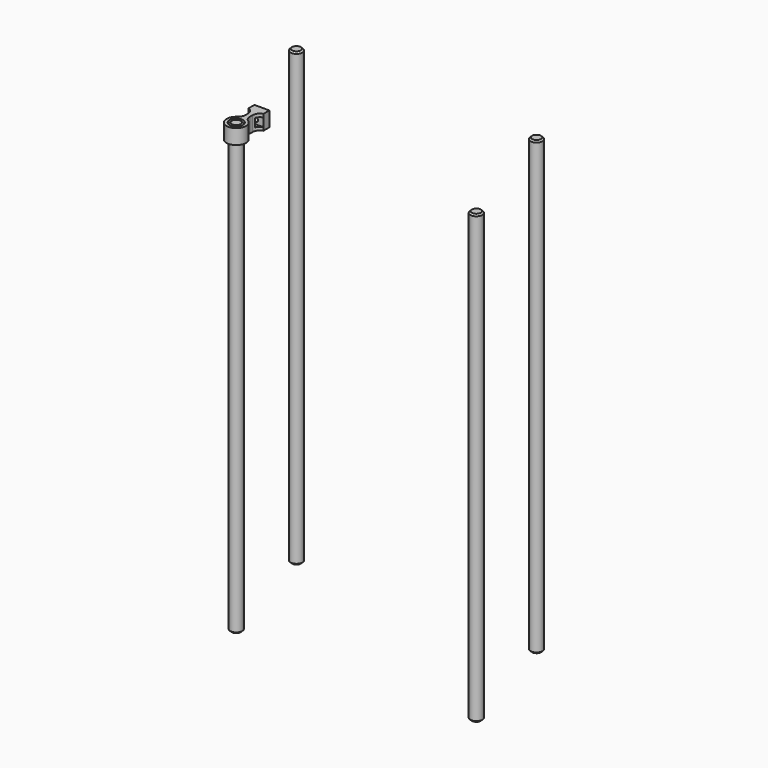
from build123d import *

# Parameters (mm, degrees)
F0_R          = 4
F1_DEPTH      = 303
F2_SIZE       = 1
F2_2_SIZE     = 1
F3_R          = 4
F4_DEPTH      = 280
F4_DEPTH_BACK = 20
F5_SIZE       = 1
F5_2_SIZE     = 1
F6_R          = 4.5
F7_DEPTH      = 10
F9_W          = 3
F9_H          = 5.7
F10_DEPTH     = 3
F8_R          = 1.5
F11_DEPTH     = 7
F12_T1_DEPTH  = 2.15
F12_T3_DEPTH  = 10
F12_T8_DEPTH  = 25.9984800354
F12_T15_DEPTH = 25.9984800354
F12_T21_DEPTH = 25.9984800354
F12_T28_DEPTH = 25.9984800354


# Not quite as in the source:
# - a fillet or chamfer that OpenCascade refuses, or shapes differently, is made with other operations: its cross-section is extruded or revolved along the edge and cut away or added


with BuildPart() as f1:
    # F0 (on Top) → F1 (new body)
    with BuildSketch(Plane.XY):
        with Locations((-80.5, 0)):
            Circle(F0_R)
    extrude(amount=F1_DEPTH)

    # F2
    f2_edges = [f1.edges().sort_by_distance(p)[0] for p in [
        (-84.5, 0, 0),
        (-84.5, 0, 303),
    ]]
    chamfer(f2_edges, length=F2_SIZE)


with BuildPart() as f1b:
    # F0 (on Top) → F1, piece 2 (new body)
    with BuildSketch(Plane.XY):
        with Locations((80.5, 0)):
            Circle(F0_R)
    extrude(amount=F1_DEPTH)

    # F2#2
    f2_2_edges = [f1b.edges().sort_by_distance(p)[0] for p in [
        (76.5, 0, 0),
        (76.5, 0, 303),
    ]]
    chamfer(f2_2_edges, length=F2_2_SIZE)


with BuildPart() as f4:
    # F3 (on Top) → F4 (new body, two sides)
    with BuildSketch(Plane.XY) as f4_sk:
        with Locations((-80.5, -50.5)):
            Circle(F3_R)
    extrude(amount=F4_DEPTH)
    extrude(f4_sk.sketch, amount=-F4_DEPTH_BACK)

    # F5
    f5_edges = [f4.edges().sort_by_distance(p)[0] for p in [
        (-84.5, -50.5, 280),
        (-84.5, -50.5, -20),
    ]]
    chamfer(f5_edges, length=F5_SIZE)


with BuildPart() as f4b:
    # F3 (on Top) → F4, piece 2 (new body, two sides)
    with BuildSketch(Plane.XY) as f4_2_sk:
        with Locations((80.5, -50.5)):
            Circle(F3_R)
    extrude(amount=F4_DEPTH)
    extrude(f4_2_sk.sketch, amount=-F4_DEPTH_BACK)

    # F5#2
    f5_2_edges = [f4b.edges().sort_by_distance(p)[0] for p in [
        (76.5, -50.5, 280),
        (76.5, -50.5, -20),
    ]]
    chamfer(f5_2_edges, length=F5_2_SIZE)


with BuildPart() as f7:
    # F6 (on face) → F7 (new body)
    with BuildSketch(Plane.XY.offset(280)):
        with BuildLine():
            Line((-82, -34), (-82, -44.1754446797))
            ThreePointArc((-82, -44.1754446797), (-80.5, -57), (-79, -44.1754446797))
            Line((-79, -44.1754446797), (-79, -34))
            Line((-79, -34), (-75.5, -34))
            Line((-75.5, -34), (-75.5, -29))
            Line((-75.5, -29), (-85.5, -29))
            Line((-85.5, -29), (-85.5, -34))
            Line((-85.5, -34), (-82, -34))
        make_face()
        with Locations((-80.5, -50.5)):
            Circle(F6_R, mode=Mode.SUBTRACT)
    extrude(amount=-F7_DEPTH)

    # F9 (on face) → F10 (cut, through all)
    with BuildSketch(Plane.YZ.offset(-79)):
        with Locations((-35.5, 275)):
            Rectangle(F9_W, F9_H)
    extrude(amount=-F10_DEPTH, mode=Mode.SUBTRACT)

    # F8 (on face) → F11 (cut)
    with BuildSketch(Plane(origin=(0, -29, 0), x_dir=(-1, 0, 0), z_dir=(0, 1, 0))):
        with Locations((80.5, 275)):
            Circle(F8_R)
    extrude(amount=-F11_DEPTH, mode=Mode.SUBTRACT)

    # F12: fillet of radius 5 on 4 edges, made by hand

    # F12_s2 → F12_t1 (join)
    with BuildSketch(Plane.XY.offset(277.85)):
        with BuildLine():
            ThreePointArc((-75.5, -34), (-78.0311288741, -35.8116561155), (-79, -38.7696960071))
            Line((-79, -38.7696960071), (-79, -34))
            Line((-79, -34), (-75.5, -34))
        make_face()
        with BuildLine():
            ThreePointArc((-85.5, -34), (-82.9688711259, -35.8116561155), (-82, -38.7696960071))
            Line((-82, -38.7696960071), (-82, -34))
            Line((-82, -34), (-85.5, -34))
        make_face()
    extrude(amount=F12_T1_DEPTH)

    # F12_s4 → F12_t3 (join)
    with BuildSketch(Plane.XY.offset(270)):
        with BuildLine():
            ThreePointArc((-79, -41.0131670195), (-78.4232586846, -43.3444290401), (-76.8260869565, -45.137877011))
            ThreePointArc((-76.8260869565, -45.137877011), (-77.8686670596, -44.5564247328), (-79, -44.1754446797))
            Line((-79, -44.1754446797), (-79, -41.0131670195))
        make_face()
        with BuildLine():
            ThreePointArc((-82, -41.0131670195), (-82.5767413154, -43.3444290401), (-84.1739130435, -45.137877011))
            ThreePointArc((-84.1739130435, -45.137877011), (-83.1313329404, -44.5564247328), (-82, -44.1754446797))
            Line((-82, -44.1754446797), (-82, -41.0131670195))
        make_face()
    extrude(amount=F12_T3_DEPTH)


with BuildPart() as f12_tool6:
    # F12_s7 → F12_t8 (new body)
    with BuildSketch(Plane.XY.offset(291.9242400177)):
        with BuildLine():
            ThreePointArc((-75.5, -34), (-78.0311288741, -35.8116561155), (-79, -38.7696960071))
            Line((-79, -38.7696960071), (-79, -34))
            Line((-79, -34), (-75.5, -34))
        make_face()
    extrude(amount=-F12_T8_DEPTH)

    split(bisect_by=Plane.XY.offset(270), keep=Keep.TOP)

    split(bisect_by=Plane.XY.offset(277.85), keep=Keep.BOTTOM)

    split(bisect_by=Plane.XZ.offset(37), keep=Keep.TOP)


with BuildPart() as f7_1:
    add(f7.part)

    # F12_t5: union F12_tool6
    add(f12_tool6.part)


with BuildPart() as f12_tool13:
    # F12_s14 → F12_t15 (new body)
    with BuildSketch(Plane.XY.offset(291.9242400177)):
        with BuildLine():
            ThreePointArc((-75.5, -34), (-78.0311288741, -35.8116561155), (-79, -38.7696960071))
            Line((-79, -38.7696960071), (-79, -34))
            Line((-79, -34), (-75.5, -34))
        make_face()
    extrude(amount=-F12_T15_DEPTH)

    split(bisect_by=Plane.XY.offset(270), keep=Keep.TOP)

    split(bisect_by=Plane.XY.offset(272.15), keep=Keep.BOTTOM)


with BuildPart() as f7_2:
    add(f7_1.part)

    # F12_t12: union F12_tool13
    add(f12_tool13.part)


with BuildPart() as f12_tool19:
    # F12_s20 → F12_t21 (new body)
    with BuildSketch(Plane.XY.offset(291.9242400177)):
        with BuildLine():
            ThreePointArc((-85.5, -34), (-82.9688711259, -35.8116561155), (-82, -38.7696960071))
            Line((-82, -38.7696960071), (-82, -34))
            Line((-82, -34), (-85.5, -34))
        make_face()
    extrude(amount=-F12_T21_DEPTH)

    split(bisect_by=Plane.XY.offset(270), keep=Keep.TOP)

    split(bisect_by=Plane.XY.offset(277.85), keep=Keep.BOTTOM)

    split(bisect_by=Plane.XZ.offset(37), keep=Keep.TOP)


with BuildPart() as f7_3:
    add(f7_2.part)

    # F12_t18: union F12_tool19
    add(f12_tool19.part)


with BuildPart() as f12_tool26:
    # F12_s27 → F12_t28 (new body)
    with BuildSketch(Plane.XY.offset(291.9242400177)):
        with BuildLine():
            ThreePointArc((-85.5, -34), (-82.9688711259, -35.8116561155), (-82, -38.7696960071))
            Line((-82, -38.7696960071), (-82, -34))
            Line((-82, -34), (-85.5, -34))
        make_face()
    extrude(amount=-F12_T28_DEPTH)

    split(bisect_by=Plane.XY.offset(270), keep=Keep.TOP)

    split(bisect_by=Plane.XY.offset(272.15), keep=Keep.BOTTOM)


with BuildPart() as f7_4:
    add(f7_3.part)

    # F12_t25: union F12_tool26
    add(f12_tool26.part)


solid = Compound([f1.part, f1b.part, f4.part, f4b.part, f7_4.part])
